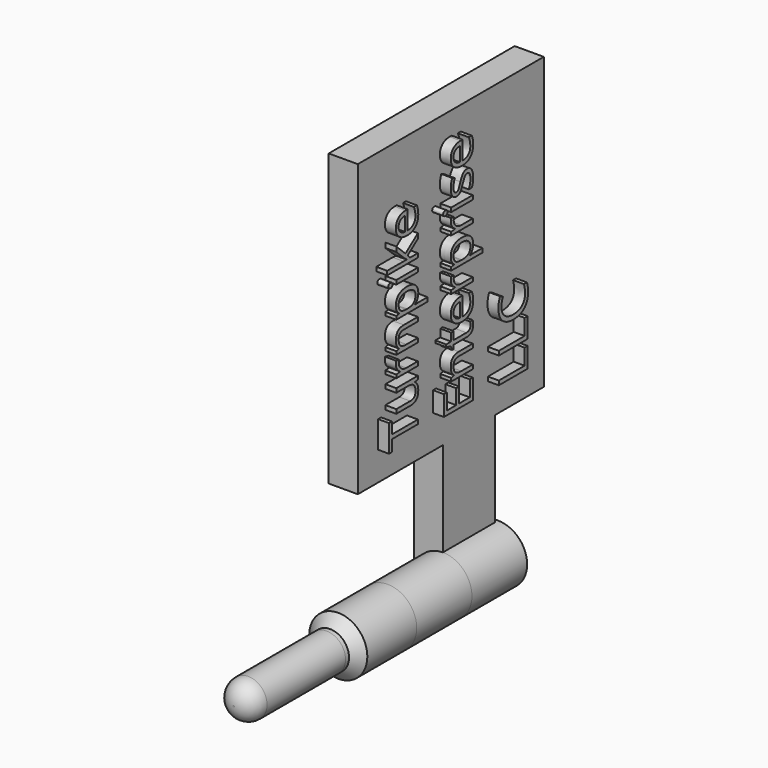
from build123d import *

# Parameters (mm, degrees)
F0_W         = 9
F0_H         = 17
F1_DEPTH     = 4
F2_R         = 2.6
F3_DEPTH     = 36
F4_R         = 4
F5_DEPTH     = 9.5
F6_R         = 4
F7_DEPTH     = 20
F8_TEXT_SIZE = 6.9444444444
F9_DEPTH     = 1.5
F10_S5_R     = 2.6
F10_T6_DEPTH = 7
F11_R        = 2.5


# Not quite as in the source:
# - a fillet or chamfer that OpenCascade refuses, or shapes differently, is made with other operations: its cross-section is extruded or revolved along the edge and cut away or added
# - Text() gives the source's letters only with a copy of the font that has no kerning and outlines rounded to 1/6400 em; it was checked with that copy


with BuildPart() as f1:
    # F0 (on Right) → F1 (new body)
    with BuildSketch(Plane.YZ):
        with Locations((4.5, 8.5)):
            Rectangle(F0_W, F0_H)
        Polygon((0, 17), (9, 17), (17.3563141078, 17), (17.3563141078, 57), (-14.6436858922, 57), (-14.6436858922, 17), align=None)
    extrude(amount=-F1_DEPTH)

    # F2 (on Front) → F3 (join)
    with BuildSketch(Plane.XZ):
        Circle(F2_R)
    extrude(amount=F3_DEPTH)

    # F4 (on Front) → F5 (join, symmetric)
    with BuildSketch(Plane.XZ):
        Circle(F4_R)
    extrude(amount=F5_DEPTH, both=True)

    # F6 (on Front) → F7 (join)
    with BuildSketch(Plane.XZ):
        Circle(F6_R)
    extrude(amount=F7_DEPTH)

    # F8 (on Right) → F9 (join)
    with BuildSketch(Plane.YZ):
        with Locations(Location((-6.1811978622, 20.9044009748), (0, 0, 90))):
            Text('Turnpike', F8_TEXT_SIZE, font='Open Sans', text_align=(TextAlign.LEFT, TextAlign.BOTTOM))
        with Locations(Location((3.2632465823, 20.9044009748), (0, 0, 90))):
            Text('Enterprise', F8_TEXT_SIZE, font='Open Sans', text_align=(TextAlign.LEFT, TextAlign.BOTTOM))
        with Locations(Location((12.7076910267, 20.9044009748), (0, 0, 90))):
            Text('LLC', F8_TEXT_SIZE, font='Open Sans', text_align=(TextAlign.LEFT, TextAlign.BOTTOM))
    extrude(amount=F9_DEPTH)

    # F10: chamfer of 2 on 1 edges, made by hand


with BuildPart() as f10_tool2:
    # F10_s3 → F10_t4 (revolve)
    with BuildSketch(Plane.XY):
        Polygon((4, -18), (2, -20), (4, -20), align=None)
    revolve(axis=Axis((0, -20, 0), (0, -1, 0)))

    # F10_s5 → F10_t6 (cut, symmetric)
    with BuildSketch(Plane.XZ.offset(19)):
        Circle(F10_S5_R)
    extrude(amount=F10_T6_DEPTH, both=True, mode=Mode.SUBTRACT)


with BuildPart() as f1_1:
    add(f1.part)

    # F10_t1: cut F10_tool2
    add(f10_tool2.part, mode=Mode.SUBTRACT)

    # F11
    f11_edges = [f1_1.edges().sort_by_distance(p)[0] for p in [
        (-2.6, -36, 0),
    ]]
    fillet(f11_edges, radius=F11_R)


solid = f1_1.part
